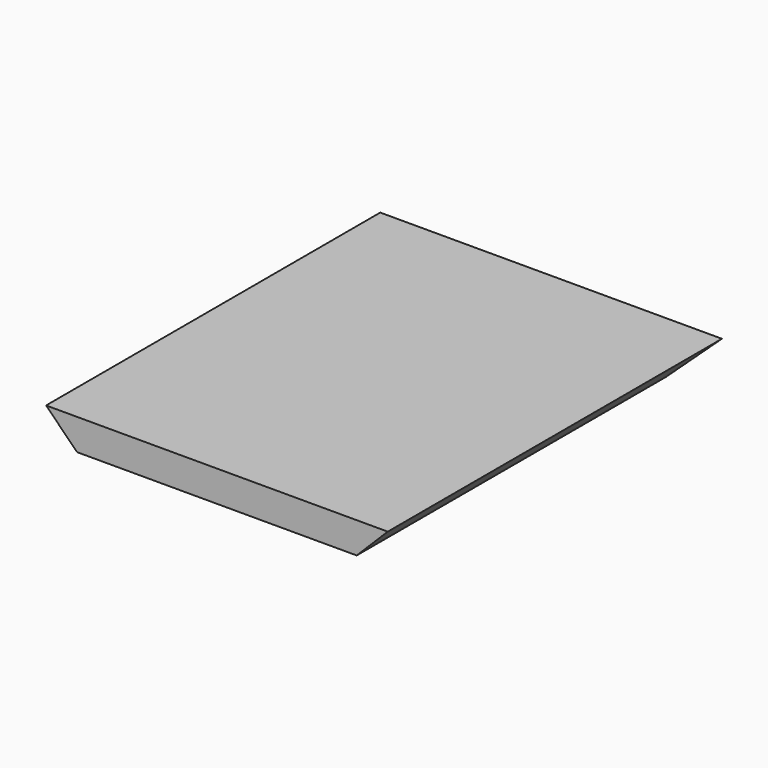
from build123d import *

# Parameters (mm, degrees)
F1_DEPTH = 5
F2_SIZE  = 4.99999


# Not quite as in the source:
# - a fillet or chamfer is up to 0.001 mm smaller than in the source, because OpenCascade refuses the exact size


with BuildPart() as f1:
    # F0 (on Top) → F1 (new body)
    with BuildSketch(Plane.XY):
        Polygon((-27.5, -11.5), (27.5, -14.74), (27.5, 52.5), (-27.5, 52.5), align=None)
        Polygon((-27.5, -14.74), (27.5, -14.74), (-27.5, -11.5), align=None)
    extrude(amount=F1_DEPTH)

    # F2 (size 5 in the source; OpenCascade refuses exactly that, so slightly less here)
    f2_edges = [f1.edges().sort_by_distance(p)[0] for p in [
        (27.5, 18.88, 0),
        (0, 52.5, 0),
        (-27.5, 18.88, 0),
    ]]
    chamfer(f2_edges, length=F2_SIZE)


solid = f1.part
